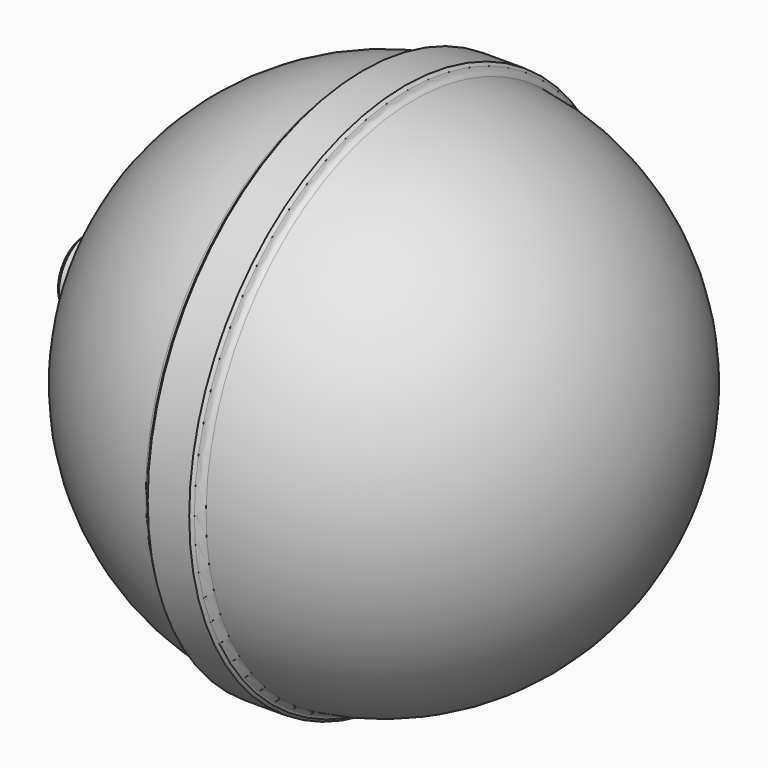
from build123d import *

# Parameters (mm, degrees)
F2_R     = 2.54
F4_D     = 14.6812
F4_DEPTH = 12.7
F4_TIP   = 4.41067746
F5_SIZE  = 1.27
F6_SIZE  = 0.762


# Not quite as in the source:
# - a fillet or chamfer that OpenCascade refuses, or shapes differently, is made with other operations: its cross-section is extruded or revolved along the edge and cut away or added


with BuildPart() as f1:
    # F0 (on Front) → F1 (revolve)
    with BuildSketch(Plane.XZ):
        with BuildLine():
            ThreePointArc((-69.7489041133, -10.16), (-70.3007351719, -5.093315157), (-70.485, 0))
            Line((-70.485, 0), (-80.645, 0))
            Line((-80.645, 0), (-80.645, -10.16))
            Line((-80.645, -10.16), (-69.7489041133, -10.16))
        make_face()
        with BuildLine():
            ThreePointArc((69.215, 0), (0, -69.215), (-69.215, 0))
            Line((-69.215, 0), (-70.485, 0))
            ThreePointArc((-70.485, 0), (-70.3007351719, -5.093315157), (-69.7489041133, -10.16))
            ThreePointArc((-69.7489041133, -10.16), (-48.4655816688, -51.1783413028), (-6.35, -70.1983812135))
            ThreePointArc((-6.35, -70.1983812135), (-3.1782326193, -70.4133088444), (0, -70.485))
            ThreePointArc((0, -70.485), (3.1782326193, -70.4133088444), (6.35, -70.1983812135))
            ThreePointArc((6.35, -70.1983812135), (52.0370780069, -47.5423783324), (70.485, 0))
            Line((70.485, 0), (69.215, 0))
        make_face()
        with BuildLine():
            ThreePointArc((0, -70.485), (-3.1782326193, -70.4133088444), (-6.35, -70.1983812135))
            Line((-6.35, -70.1983812135), (-6.35, -72.517))
            Line((-6.35, -72.517), (0, -72.517))
            Line((0, -72.517), (0, -70.485))
        make_face()
        with BuildLine():
            Line((6.35, -72.517), (6.35, -70.1983812135))
            ThreePointArc((6.35, -70.1983812135), (3.1782326193, -70.4133088444), (0, -70.485))
            Line((0, -70.485), (0, -72.517))
            Line((0, -72.517), (6.35, -72.517))
        make_face()
    revolve(axis=Axis((-35.2425, 0, 0), (-1, 0, 0)))

    # F2
    f2_edges = [f1.edges().sort_by_distance(p)[0] for p in [
        (-69.748904, 0, 10.16),
    ]]
    fillet(f2_edges, radius=F2_R)

    # F4
    with Locations(Plane(origin=(-80.645, 0, 0), x_dir=(0, -1, 0), z_dir=(-1, 0, 0))):
        with Locations((0, 0)):
            Hole(F4_D / 2, depth=F4_DEPTH)
            with Locations((0, 0, -(F4_DEPTH + F4_TIP / 2))):  # 118° drill point
                Cone(0, F4_D / 2, F4_TIP, mode=Mode.SUBTRACT)

    # F5
    f5_edges = [f1.edges().sort_by_distance(p)[0] for p in [
        (-80.645, 0, 10.16),
    ]]
    chamfer(f5_edges, length=F5_SIZE)

    # F6
    f6_edges = [f1.edges().sort_by_distance(p)[0] for p in [
        (-6.35, 0, 72.517),
        (6.35, 0, 72.517),
    ]]
    chamfer(f6_edges, length=F6_SIZE)

    # F7: fillet of radius 2.032 on 2 edges, made by hand

    # F7_s1 → F7_t2 (revolve)
    with BuildSketch(Plane.XZ):
        with BuildLine():
            ThreePointArc((-6.35, -71.755), (-6.9417364445, -70.5807921178), (-8.1285337342, -70.0147281958))
            ThreePointArc((-8.1285337342, -70.0147281958), (-7.2398492305, -70.1121944323), (-6.35, -70.1983812135))
            Line((-6.35, -70.1983812135), (-6.35, -71.755))
        make_face()
    revolve(axis=Axis((-6.35, 0, 0), (-1, 0, 0)))

    # F7_s3 → F7_t4 (revolve)
    with BuildSketch(Plane.XZ):
        with BuildLine():
            ThreePointArc((6.35, -71.755), (6.9417364445, -70.5807921178), (8.1285337342, -70.0147281958))
            ThreePointArc((8.1285337342, -70.0147281958), (7.2398492305, -70.1121944323), (6.35, -70.1983812135))
            Line((6.35, -70.1983812135), (6.35, -71.755))
        make_face()
    revolve(axis=Axis((6.35, 0, 0), (-1, 0, 0)))


solid = f1.part
